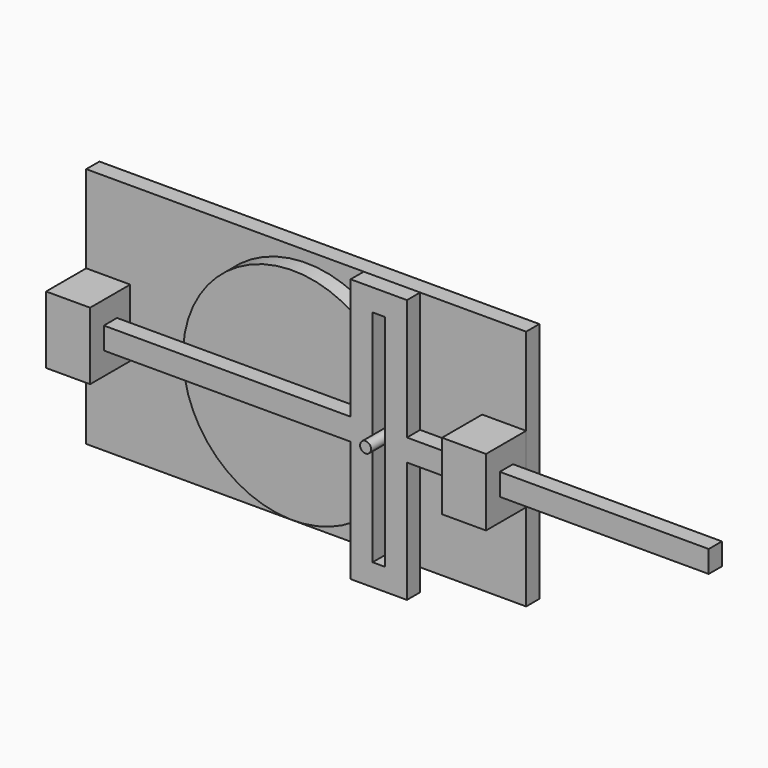
from build123d import *

# Parameters (mm, degrees)
F2_R      = 63.5
F2_R_2    = 3.571875
F3_DEPTH  = 9.525
F4_R      = 3.175
F5_DEPTH  = 19.05
F6_W      = 12.7
F6_H      = 12.7
F6_W_2    = 174.228125
F7_DEPTH  = 9.525
F8_W      = 254
F8_H      = 139.7
F9_DEPTH  = 9.525
F11_DEPTH = 28.971875


# Not quite as in the source:
# - a length typed as a fraction of an inch, garbled in the dataset ("3 / 203.2 mm" for 3/8 in), is restored


with BuildPart() as f3:
    # F2 (on Front) → F3 (new body)
    with BuildSketch(Plane.XZ):
        Circle(F2_R)
        Circle(F2_R_2, mode=Mode.SUBTRACT)
    extrude(amount=F3_DEPTH)

    # F4 (on face) → F5 (join)
    with BuildSketch(Plane.XZ.offset(9.525)):
        with Locations((57.15, 0)):
            Circle(F4_R)
    extrude(amount=F5_DEPTH)

    # F8 (on Front) → F9 (join)
    with BuildSketch(Plane.XZ):
        Rectangle(F8_W, F8_H)
    extrude(amount=-F9_DEPTH)


with BuildPart() as f7:
    # F6 (on face) → F7 (new body)
    with BuildSketch(Plane.XZ.offset(9.525)):
        Polygon((53.578125, 63.5), (60.721875, 63.5), (60.721875, 6.35), (73.421875, 6.35), (73.421875, 76.2), (40.878125, 76.2), (40.878125, 6.35), (53.578125, 6.35), align=None)
        with Locations((67.071875, 0)):
            Rectangle(F6_W, F6_H)
        with Locations((47.228125, 0)):
            Rectangle(F6_W, F6_H)
        Polygon((73.421875, -6.35), (60.721875, -6.35), (60.721875, -63.5), (53.578125, -63.5), (53.578125, -6.35), (40.878125, -6.35), (40.878125, -76.2), (73.421875, -76.2), align=None)
        with Locations((160.5359375, 0)):
            Rectangle(F6_W_2, F6_H)
        with Locations((-46.2359375, 0)):
            Rectangle(F6_W_2, F6_H)
    extrude(amount=F7_DEPTH)


with BuildPart() as f11:
    # F10 (on face) → F11 (new body)
    with BuildSketch(Plane.XZ):
        Polygon((-127, 19.446875), (-127, 0), (-127, -19.446875), (-101.6, -19.446875), (-101.6, 19.446875), align=None)
    extrude(amount=F11_DEPTH)


with BuildPart() as f11b:
    # F10 (on face) → F11, piece 2 (new body)
    with BuildSketch(Plane.XZ):
        Polygon((127, 0), (127, 19.446875), (101.6, 19.446875), (101.6, -19.446875), (127, -19.446875), align=None)
    extrude(amount=F11_DEPTH)


solid = Compound([f3.part, f7.part, f11.part, f11b.part])
